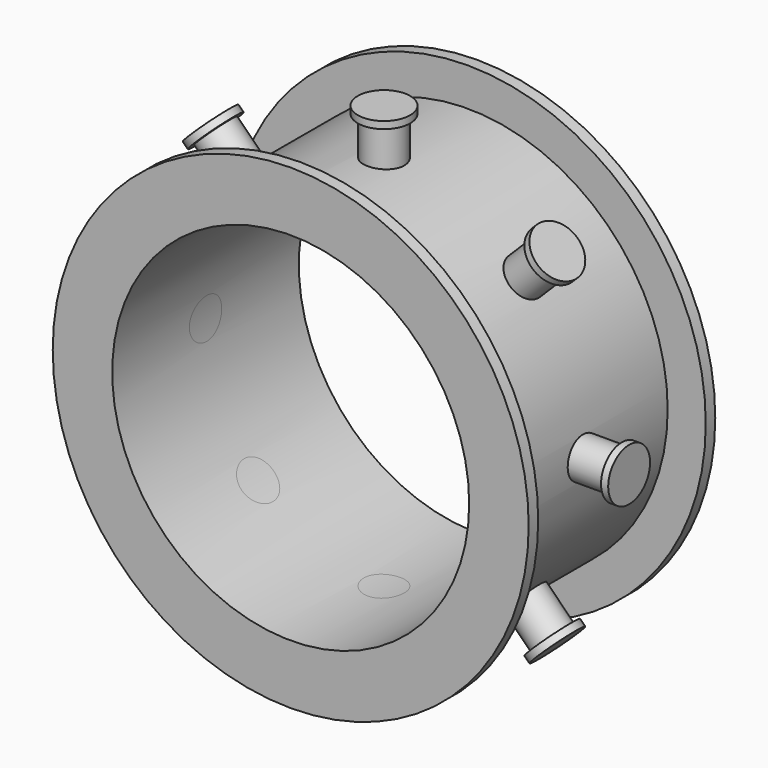
from build123d import *

# Parameters (mm, degrees)
F0_R            = 12.7
F0_R_2          = 9.525
F1_DEPTH        = 6.223
F2_R            = 15.24
F2_R_2          = 10.668
F3_DEPTH        = 5.588
F4_R            = 1.0795
F6_DEPTH        = 12.7
F6_COPIES_COUNT = 8
F7_R            = 1.397
F8_DEPTH        = 0.381
F8_COPIES_COUNT = 8
F9_R            = 9.525
F10_DEPTH       = 12.4470001


# Not quite as in the source:
# - a pattern or mirror of a feature is missing from the dataset's text; its kind, count and spacing are read off the source's solid


with BuildPart() as f1:
    # F0 (on Front) → F1 (new body, symmetric)
    with BuildSketch(Plane.XZ):
        Circle(F0_R)
        Circle(F0_R_2, mode=Mode.SUBTRACT)
    extrude(amount=F1_DEPTH, both=True)

    # F2 (on Front) → F3 (cut, symmetric)
    with BuildSketch(Plane.XZ):
        Circle(F2_R)
        Circle(F2_R_2, mode=Mode.SUBTRACT)
    extrude(amount=F3_DEPTH, both=True, mode=Mode.SUBTRACT)

    # F4 (on Right) → F6 (join)
    with BuildSketch(Plane.YZ):
        Circle(F4_R)
    f6 = extrude(amount=-F6_DEPTH)

    # F6_copies: F6 ×8 about axis
    f6_copies_axis = Axis((0, 0, 0), (0, 1, 0))
    for i in range(1, F6_COPIES_COUNT):
        add(f6.rotate(f6_copies_axis, i * 360 / F6_COPIES_COUNT))

    # F7 (on face) → F8 (join)
    with BuildSketch(Plane(origin=(-12.7, 0, 0), x_dir=(0, -1, 0), z_dir=(-1, 0, 0))):
        Circle(F7_R)
    f8 = extrude(amount=F8_DEPTH)

    # F8_copies: F8 ×8 about axis
    f8_copies_axis = Axis((0, 0, 0), (0, 1, 0))
    for i in range(1, F8_COPIES_COUNT):
        add(f8.rotate(f8_copies_axis, i * 360 / F8_COPIES_COUNT))

    # F9 (on face) → F10 (cut, through all)
    with BuildSketch(Plane.XZ.offset(6.223)):
        Circle(F9_R)
    extrude(amount=-F10_DEPTH, mode=Mode.SUBTRACT)


solid = f1.part
